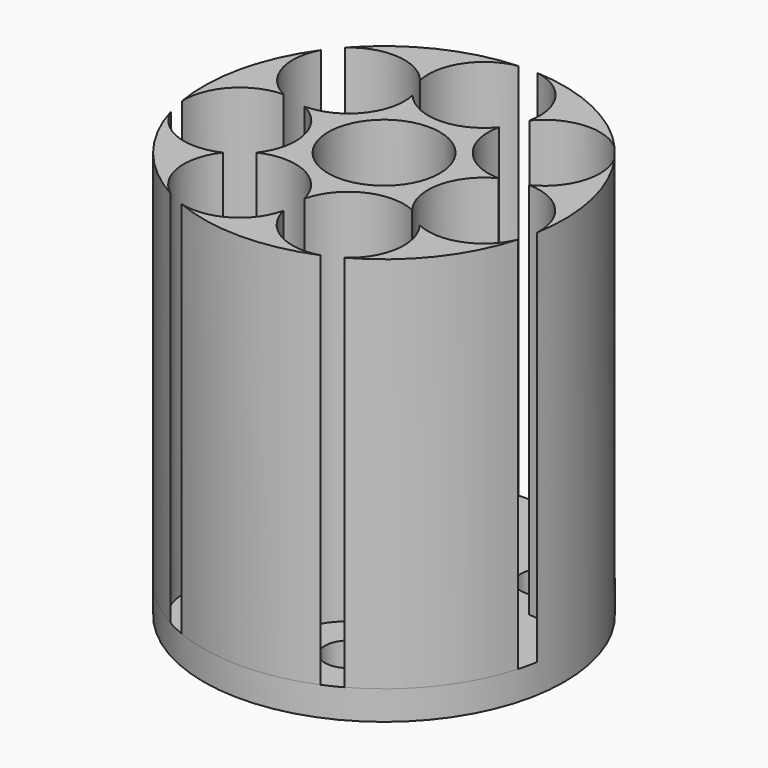
from build123d import *

# Parameters (mm, degrees)
F1_DEPTH = 65
F0_R     = 9.6
F2_R     = 31
F2_R_2   = 9.6
F3_DEPTH = 5
F5_D     = 8


with BuildPart() as f1:
    # F0 (on Top) → F1 (new body)
    with BuildSketch(Plane.XY):
        with BuildLine():
            ThreePointArc((0, -21.6377846635), (-4.4866514155, -27.6603721731), (-11.936497657, -28.6097889486))
            ThreePointArc((-11.936497657, -28.6097889486), (0, -31), (11.936497657, -28.6097889486))
            ThreePointArc((11.936497657, -28.6097889486), (4.4866514155, -27.6603721731), (0, -21.6377846635))
        make_face()
    extrude(amount=F1_DEPTH)



with BuildPart() as f1b:
    # F0 (on Top) → F1, piece 2 (new body)
    with BuildSketch(Plane.XY):
        with BuildLine():
            ThreePointArc((7.421093957, 15.4100603877), (0, 11.9), (-7.421093957, 15.4100603877))
            ThreePointArc((-7.421093957, 15.4100603877), (-9.3037946414, 7.4195286421), (-16.6750467587, 3.8059706078))
            ThreePointArc((-16.6750467587, 3.8059706078), (-11.601642155, -2.6479991141), (-13.3723492421, -10.6640926674))
            ThreePointArc((-13.3723492421, -10.6640926674), (-5.1632164955, -10.721529528), (0, -17.1038766563))
            ThreePointArc((0, -17.1038766563), (5.1632164955, -10.721529528), (13.3723492421, -10.6640926674))
            ThreePointArc((13.3723492421, -10.6640926674), (11.601642155, -2.6479991141), (16.6750467587, 3.8059706078))
            ThreePointArc((16.6750467587, 3.8059706078), (9.3037946414, 7.4195286421), (7.421093957, 15.4100603877))
        make_face()
        Circle(F0_R, mode=Mode.SUBTRACT)
    extrude(amount=F1_DEPTH)


with BuildPart() as f1c:
    # F0 (on Top) → F1, piece 3 (new body)
    with BuildSketch(Plane.XY):
        with BuildLine():
            ThreePointArc((-23.1677349851, 20.5974769246), (-16.0437189504, 22.9744491102), (-9.388282916, 19.4949703522))
            ThreePointArc((-9.388282916, 19.4949703522), (-7.9590524573, 26.8678192948), (-1.6589094237, 30.9555813953))
            ThreePointArc((-1.6589094237, 30.9555813953), (-13.4503959126, 27.930034905), (-23.1677349851, 20.5974769246))
        make_face()
    extrude(amount=F1_DEPTH)


with BuildPart() as f1d:
    # F0 (on Top) → F1, piece 4 (new body)
    with BuildSketch(Plane.XY):
        with BuildLine():
            ThreePointArc((-30.5486024144, -5.2709477823), (-27.9652427562, 1.7808501523), (-21.0952802263, 4.8148600521))
            ThreePointArc((-21.0952802263, 4.8148600521), (-25.9684950295, 10.5291735468), (-25.2363612008, 18.0035016966))
            ThreePointArc((-25.2363612008, 18.0035016966), (-30.2227652776, 6.8981489526), (-30.5486024144, -5.2709477823))
        make_face()
    extrude(amount=F1_DEPTH)


with BuildPart() as f1e:
    # F0 (on Top) → F1, piece 5 (new body)
    with BuildSketch(Plane.XY):
        with BuildLine():
            ThreePointArc((-14.9257491478, -27.1702413014), (-18.8283683796, -20.7537652931), (-16.9171012608, -13.4909380725))
            ThreePointArc((-16.9171012608, -13.4909380725), (-24.4231311838, -13.738154638), (-29.8103182658, -8.5055819842))
            ThreePointArc((-29.8103182658, -8.5055819842), (-24.2367759565, -19.3281838576), (-14.9257491478, -27.1702413014))
        make_face()
    extrude(amount=F1_DEPTH)


with BuildPart() as f1f:
    # F0 (on Top) → F1, piece 6 (new body)
    with BuildSketch(Plane.XY):
        with BuildLine():
            ThreePointArc((29.8103182658, -8.5055819842), (24.4231311838, -13.738154638), (16.9171012608, -13.4909380725))
            ThreePointArc((16.9171012608, -13.4909380725), (18.8283683796, -20.7537652931), (14.9257491478, -27.1702413014))
            ThreePointArc((14.9257491478, -27.1702413014), (24.2367759565, -19.3281838576), (29.8103182658, -8.5055819842))
        make_face()
    extrude(amount=F1_DEPTH)


with BuildPart() as f1g:
    # F0 (on Top) → F1, piece 7 (new body)
    with BuildSketch(Plane.XY):
        with BuildLine():
            ThreePointArc((25.2363612008, 18.0035016966), (25.9684950295, 10.5291735468), (21.0952802263, 4.8148600521))
            ThreePointArc((21.0952802263, 4.8148600521), (27.9652427562, 1.7808501523), (30.5486024144, -5.2709477823))
            ThreePointArc((30.5486024144, -5.2709477823), (30.2227652776, 6.8981489526), (25.2363612008, 18.0035016966))
        make_face()
    extrude(amount=F1_DEPTH)


with BuildPart() as f1h:
    # F0 (on Top) → F1, piece 8 (new body)
    with BuildSketch(Plane.XY):
        with BuildLine():
            ThreePointArc((1.6589094237, 30.9555813953), (7.9590524573, 26.8678192948), (9.388282916, 19.4949703522))
            ThreePointArc((9.388282916, 19.4949703522), (16.0437189504, 22.9744491102), (23.1677349851, 20.5974769246))
            ThreePointArc((23.1677349851, 20.5974769246), (13.4503959126, 27.930034905), (1.6589094237, 30.9555813953))
        make_face()
    extrude(amount=F1_DEPTH)


with BuildPart() as f1_1:
    add(f1.part)

    add(f1b.part)  # F3 merges F1b

    add(f1c.part)  # F3 merges F1c

    add(f1d.part)  # F3 merges F1d

    add(f1e.part)  # F3 merges F1e

    add(f1f.part)  # F3 merges F1f

    add(f1g.part)  # F3 merges F1g

    add(f1h.part)  # F3 merges F1h
    # F2 (on face) → F3 (join)
    with BuildSketch(Plane(origin=(0, 0, 0), x_dir=(1, 0, 0), z_dir=(0, 0, -1))):
        Circle(F2_R)
        with BuildLine():
            ThreePointArc((-13.3723492421, 10.6640926674), (-5.1632164955, 10.721529528), (0, 17.1038766563))
            ThreePointArc((0, 17.1038766563), (5.1632164955, 10.721529528), (13.3723492421, 10.6640926674))
            ThreePointArc((13.3723492421, 10.6640926674), (11.601642155, 2.6479991141), (16.6750467587, -3.8059706078))
            ThreePointArc((16.6750467587, -3.8059706078), (9.3037946414, -7.4195286421), (7.421093957, -15.4100603877))
            ThreePointArc((7.421093957, -15.4100603877), (0, -11.9), (-7.421093957, -15.4100603877))
            ThreePointArc((-7.421093957, -15.4100603877), (-9.3037946414, -7.4195286421), (-16.6750467587, -3.8059706078))
            ThreePointArc((-16.6750467587, -3.8059706078), (-11.601642155, 2.6479991141), (-13.3723492421, 10.6640926674))
        make_face(mode=Mode.SUBTRACT)
        with BuildLine():
            ThreePointArc((13.3723492421, 10.6640926674), (5.1632164955, 10.721529528), (0, 17.1038766563))
            ThreePointArc((0, 17.1038766563), (-5.1632164955, 10.721529528), (-13.3723492421, 10.6640926674))
            ThreePointArc((-13.3723492421, 10.6640926674), (-11.601642155, 2.6479991141), (-16.6750467587, -3.8059706078))
            ThreePointArc((-16.6750467587, -3.8059706078), (-9.3037946414, -7.4195286421), (-7.421093957, -15.4100603877))
            ThreePointArc((-7.421093957, -15.4100603877), (0, -11.9), (7.421093957, -15.4100603877))
            ThreePointArc((7.421093957, -15.4100603877), (9.3037946414, -7.4195286421), (16.6750467587, -3.8059706078))
            ThreePointArc((16.6750467587, -3.8059706078), (11.601642155, 2.6479991141), (13.3723492421, 10.6640926674))
        make_face()
        Circle(F2_R_2, mode=Mode.SUBTRACT)
        Circle(F2_R_2)
    extrude(amount=F3_DEPTH)

    # F5 (through all)
    with Locations(Plane.XY):
        with Locations((9.328500391, -19.3708306599), (20.9609501119, -4.7842000801), (16.8093768731, 13.40503074), (0, 21.5), (0, 0), (-16.8093768731, 13.40503074), (-20.9609501119, -4.7842000801), (-9.328500391, -19.3708306599)):
            Hole(F5_D / 2)


solid = f1_1.part
